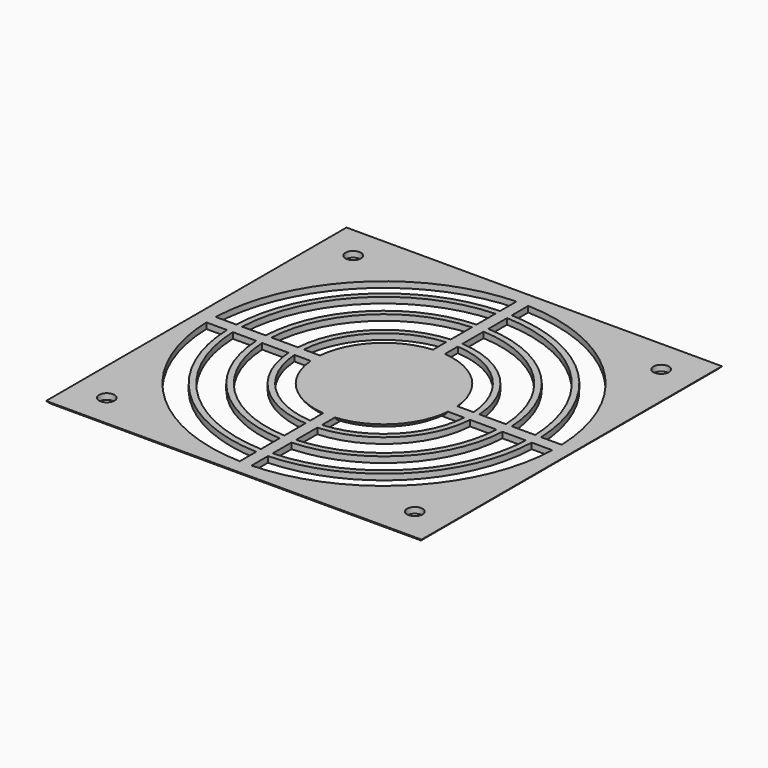
from build123d import *

# Parameters (mm, degrees)
F0_W            = 128
F0_H            = 128
F1_DEPTH        = 2
F3_DEPTH        = 25
F4_R            = 2.65
F5_DEPTH        = 25
F5_COPIES_COUNT = 4
F6_T1_DEPTH     = 148
F6_T3_DEPTH     = 148
F7_T4_ANGLE     = 122.478644554
F7_T9_ANGLE     = 122.478644554
F7_T15_ANGLE    = 122.478644554
F7_T20_ANGLE    = 122.478644554
F7_T25_ANGLE    = 122.478644554
F7_T31_ANGLE    = 122.478644554
F7_T36_ANGLE    = 122.478644554
F7_T41_ANGLE    = 122.478644554
F7_T47_ANGLE    = 122.478644554
F7_T52_ANGLE    = 122.478644554
F7_T57_ANGLE    = 122.478644554
F7_T63_ANGLE    = 122.478644554


# Not quite as in the source:
# - a fillet or chamfer that OpenCascade refuses, or shapes differently, is made with other operations: its cross-section is extruded or revolved along the edge and cut away or added
# - a pattern or mirror of a feature is missing from the dataset's text; its kind, count and spacing are read off the source's solid
# - a feature names something its author has since deleted; it is built from what else it names


with BuildPart() as f1:
    # F0 (on Top) → F1 (new body)
    with BuildSketch(Plane.XY):
        Rectangle(F0_W, F0_H)
    extrude(amount=F1_DEPTH)

    # F2 (on face) → F3 (cut)
    with BuildSketch(Plane.XY.offset(2)):
        with BuildLine():
            Line((51.9615242271, 2), (58.9660919512, 2))
            ThreePointArc((58.9660919512, 2), (41.71930009, 41.71930009), (2, 58.9660919512))
            Line((2, 58.9660919512), (2, 51.9615242271))
            ThreePointArc((2, 51.9615242271), (36.7695526217, 36.7695526217), (51.9615242271, 2))
        make_face()
        with BuildLine():
            Line((41.9523539268, 2), (49.9599839872, 2))
            ThreePointArc((49.9599839872, 2), (35.3553390593, 35.3553390593), (2, 49.9599839872))
            Line((2, 49.9599839872), (2, 41.9523539268))
            ThreePointArc((2, 41.9523539268), (29.6984848098, 29.6984848098), (41.9523539268, 2))
        make_face()
        with BuildLine():
            Line((30.9354165965, 2), (39.9499687109, 2))
            ThreePointArc((39.9499687109, 2), (28.2842712475, 28.2842712475), (2, 39.9499687109))
            Line((2, 39.9499687109), (2, 30.9354165965))
            ThreePointArc((2, 30.9354165965), (21.9203102168, 21.9203102168), (30.9354165965, 2))
        make_face()
        with BuildLine():
            Line((23.4147389479, 2), (28.930952283, 2))
            ThreePointArc((28.930952283, 2), (20.5060966544, 20.5060966544), (2, 28.930952283))
            Line((2, 28.930952283), (2, 23.4147389479))
            ThreePointArc((2, 23.4147389479), (16.6170093579, 16.6170093579), (23.4147389479, 2))
        make_face()
        with BuildLine():
            ThreePointArc((2, -28.930952283), (20.5060966544, -20.5060966544), (28.930952283, -2))
            Line((28.930952283, -2), (23.4147389479, -2))
            ThreePointArc((23.4147389479, -2), (16.6170093579, -16.6170093579), (2, -23.4147389479))
            Line((2, -23.4147389479), (2, -28.930952283))
        make_face()
        with BuildLine():
            ThreePointArc((2, -39.9499687109), (28.2842712475, -28.2842712475), (39.9499687109, -2))
            Line((39.9499687109, -2), (30.9354165965, -2))
            ThreePointArc((30.9354165965, -2), (21.9203102168, -21.9203102168), (2, -30.9354165965))
            Line((2, -30.9354165965), (2, -39.9499687109))
        make_face()
        with BuildLine():
            ThreePointArc((2, -49.9599839872), (35.3553390593, -35.3553390593), (49.9599839872, -2))
            Line((49.9599839872, -2), (41.9523539268, -2))
            ThreePointArc((41.9523539268, -2), (29.6984848098, -29.6984848098), (2, -41.9523539268))
            Line((2, -41.9523539268), (2, -49.9599839872))
        make_face()
        with BuildLine():
            ThreePointArc((2, -58.9660919512), (41.71930009, -41.71930009), (58.9660919512, -2))
            Line((58.9660919512, -2), (51.9615242271, -2))
            ThreePointArc((51.9615242271, -2), (36.7695526217, -36.7695526217), (2, -51.9615242271))
            Line((2, -51.9615242271), (2, -58.9660919512))
        make_face()
        with BuildLine():
            ThreePointArc((-28.930952283, -2), (-20.5060966544, -20.5060966544), (-2, -28.930952283))
            Line((-2, -28.930952283), (-2, -23.4147389479))
            ThreePointArc((-2, -23.4147389479), (-16.6170093579, -16.6170093579), (-23.4147389479, -2))
            Line((-23.4147389479, -2), (-28.930952283, -2))
        make_face()
        with BuildLine():
            ThreePointArc((-39.9499687109, -2), (-28.2842712475, -28.2842712475), (-2, -39.9499687109))
            Line((-2, -39.9499687109), (-2, -30.9354165965))
            ThreePointArc((-2, -30.9354165965), (-21.9203102168, -21.9203102168), (-30.9354165965, -2))
            Line((-30.9354165965, -2), (-39.9499687109, -2))
        make_face()
        with BuildLine():
            ThreePointArc((-49.9599839872, -2), (-35.3553390593, -35.3553390593), (-2, -49.9599839872))
            Line((-2, -49.9599839872), (-2, -41.9523539268))
            ThreePointArc((-2, -41.9523539268), (-29.6984848098, -29.6984848098), (-41.9523539268, -2))
            Line((-41.9523539268, -2), (-49.9599839872, -2))
        make_face()
        with BuildLine():
            ThreePointArc((-58.9660919512, -2), (-41.71930009, -41.71930009), (-2, -58.9660919512))
            Line((-2, -58.9660919512), (-2, -51.9615242271))
            ThreePointArc((-2, -51.9615242271), (-36.7695526217, -36.7695526217), (-51.9615242271, -2))
            Line((-51.9615242271, -2), (-58.9660919512, -2))
        make_face()
        with BuildLine():
            Line((-2, 23.4147389479), (-2, 28.930952283))
            ThreePointArc((-2, 28.930952283), (-20.5060966544, 20.5060966544), (-28.930952283, 2))
            Line((-28.930952283, 2), (-23.4147389479, 2))
            ThreePointArc((-23.4147389479, 2), (-16.6170093579, 16.6170093579), (-2, 23.4147389479))
        make_face()
        with BuildLine():
            Line((-2, 30.9354165965), (-2, 39.9499687109))
            ThreePointArc((-2, 39.9499687109), (-28.2842712475, 28.2842712475), (-39.9499687109, 2))
            Line((-39.9499687109, 2), (-30.9354165965, 2))
            ThreePointArc((-30.9354165965, 2), (-21.9203102168, 21.9203102168), (-2, 30.9354165965))
        make_face()
        with BuildLine():
            Line((-2, 41.9523539268), (-2, 49.9599839872))
            ThreePointArc((-2, 49.9599839872), (-35.3553390593, 35.3553390593), (-49.9599839872, 2))
            Line((-49.9599839872, 2), (-41.9523539268, 2))
            ThreePointArc((-41.9523539268, 2), (-29.6984848098, 29.6984848098), (-2, 41.9523539268))
        make_face()
        with BuildLine():
            Line((-2, 51.9615242271), (-2, 58.9660919512))
            ThreePointArc((-2, 58.9660919512), (-41.71930009, 41.71930009), (-58.9660919512, 2))
            Line((-58.9660919512, 2), (-51.9615242271, 2))
            ThreePointArc((-51.9615242271, 2), (-36.7695526217, 36.7695526217), (-2, 51.9615242271))
        make_face()
    extrude(amount=-F3_DEPTH, mode=Mode.SUBTRACT)

    # F4 (on face) → F5 (cut)
    with BuildSketch(Plane.XY.offset(2)):
        with Locations((-52.5, 52.5)):
            Circle(F4_R)
    f5 = extrude(amount=-F5_DEPTH, mode=Mode.SUBTRACT)

    # F5_copies: F5 ×4 about axis
    f5_copies_axis = Axis((0, 0, 0), (0, 0, 1))
    for i in range(1, F5_COPIES_COUNT):
        add(f5.rotate(f5_copies_axis, i * 360 / F5_COPIES_COUNT), mode=Mode.SUBTRACT)

    # F6: fillet of radius 5 on 4 edges, made by hand

    # F6_s2 → F6_t1 (cut)
    with BuildSketch(Plane.YZ.offset(-74)):
        with BuildLine():
            ThreePointArc((-60, 0), (-62.2360679775, 0.527864045), (-64, 2))
            Line((-64, 2), (-64, 0))
            Line((-64, 0), (-60, 0))
        make_face()
        with BuildLine():
            ThreePointArc((64, 2), (62.2360679775, 0.527864045), (60, 0))
            Line((60, 0), (64, 0))
            Line((64, 0), (64, 2))
        make_face()
    extrude(amount=F6_T1_DEPTH, mode=Mode.SUBTRACT)

    # F6_s4 → F6_t3 (cut)
    with BuildSketch(Plane.XZ.offset(-74)):
        with BuildLine():
            ThreePointArc((-64, 2), (-62.2360679775, 0.527864045), (-60, 0))
            Line((-60, 0), (-64, 0))
            Line((-64, 0), (-64, 2))
        make_face()
        with BuildLine():
            ThreePointArc((64, 2), (62.2360679775, 0.527864045), (60, 0))
            Line((60, 0), (64, 0))
            Line((64, 0), (64, 2))
        make_face()
    extrude(amount=F6_T3_DEPTH, mode=Mode.SUBTRACT)

    # F7: fillet of radius 4 on 4 edges, made by hand


with BuildPart() as f7_tool2:
    # F7_s3 → F7_t4 (revolve)
    with BuildSketch(Plane(origin=(0, 0, 0), x_dir=(0, 0, 1), z_dir=(0.960101987, -0.2796500929, 0))):
        with BuildLine():
            ThreePointArc((2, -23.5), (0.5358983849, -22.0358983849), (0, -20.0358983849))
            Line((0, -20.0358983849), (0, -23.5))
            Line((0, -23.5), (2, -23.5))
        make_face()
    revolve(axis=Axis((0, 0, 0), (0, 0, 1)), revolution_arc=F7_T4_ANGLE)

    split(bisect_by=Plane.YZ.offset(2), keep=Keep.TOP)


with BuildPart() as f1_1:
    add(f1.part)

    # F7_t1: cut F7_tool2
    add(f7_tool2.part, mode=Mode.SUBTRACT)


with BuildPart() as f7_tool7:
    # F7_s8 → F7_t9 (revolve)
    with BuildSketch(Plane(origin=(0, 0, 0), x_dir=(0, 0, 1), z_dir=(0.960101987, -0.2796500929, 0))):
        with BuildLine():
            ThreePointArc((2, -23.5), (0.5358983849, -22.0358983849), (0, -20.0358983849))
            Line((0, -20.0358983849), (0, -23.5))
            Line((0, -23.5), (2, -23.5))
        make_face()
    revolve(axis=Axis((0, 0, 0), (0, 0, 1)), revolution_arc=F7_T9_ANGLE)

    split(bisect_by=Plane.YZ.offset(-2), keep=Keep.BOTTOM)

    split(bisect_by=Plane.XZ.offset(-2), keep=Keep.BOTTOM)


with BuildPart() as f1_2:
    add(f1_1.part)

    # F7_t6: cut F7_tool7
    add(f7_tool7.part, mode=Mode.SUBTRACT)


with BuildPart() as f7_tool13:
    # F7_s14 → F7_t15 (revolve)
    with BuildSketch(Plane(origin=(0, 0, 0), x_dir=(0, 0, 1), z_dir=(0.960101987, -0.2796500929, 0))):
        with BuildLine():
            ThreePointArc((2, -23.5), (0.5358983849, -22.0358983849), (0, -20.0358983849))
            Line((0, -20.0358983849), (0, -23.5))
            Line((0, -23.5), (2, -23.5))
        make_face()
    revolve(axis=Axis((0, 0, 0), (0, 0, 1)), revolution_arc=F7_T15_ANGLE)

    split(bisect_by=Plane.XZ.offset(2), keep=Keep.TOP)


with BuildPart() as f1_3:
    add(f1_2.part)

    # F7_t12: cut F7_tool13
    add(f7_tool13.part, mode=Mode.SUBTRACT)


with BuildPart() as f7_tool18:
    # F7_s19 → F7_t20 (revolve)
    with BuildSketch(Plane(origin=(0, 0, 0), x_dir=(0, 0, 1), z_dir=(-0.2796500929, -0.960101987, 0))):
        with BuildLine():
            ThreePointArc((2, -23.5), (0.5358983849, -22.0358983849), (0, -20.0358983849))
            Line((0, -20.0358983849), (0, -23.5))
            Line((0, -23.5), (2, -23.5))
        make_face()
    revolve(axis=Axis((0, 0, 0), (0, 0, 1)), revolution_arc=F7_T20_ANGLE)

    split(bisect_by=Plane.XZ.offset(2), keep=Keep.TOP)


with BuildPart() as f1_4:
    add(f1_3.part)

    # F7_t17: cut F7_tool18
    add(f7_tool18.part, mode=Mode.SUBTRACT)


with BuildPart() as f7_tool23:
    # F7_s24 → F7_t25 (revolve)
    with BuildSketch(Plane(origin=(0, 0, 0), x_dir=(0, 0, 1), z_dir=(-0.2796500929, -0.960101987, 0))):
        with BuildLine():
            ThreePointArc((2, -23.5), (0.5358983849, -22.0358983849), (0, -20.0358983849))
            Line((0, -20.0358983849), (0, -23.5))
            Line((0, -23.5), (2, -23.5))
        make_face()
    revolve(axis=Axis((0, 0, 0), (0, 0, 1)), revolution_arc=F7_T25_ANGLE)

    split(bisect_by=Plane.XZ.offset(-2), keep=Keep.BOTTOM)

    split(bisect_by=Plane.YZ.offset(2), keep=Keep.TOP)


with BuildPart() as f1_5:
    add(f1_4.part)

    # F7_t22: cut F7_tool23
    add(f7_tool23.part, mode=Mode.SUBTRACT)


with BuildPart() as f7_tool29:
    # F7_s30 → F7_t31 (revolve)
    with BuildSketch(Plane(origin=(0, 0, 0), x_dir=(0, 0, 1), z_dir=(-0.2796500929, -0.960101987, 0))):
        with BuildLine():
            ThreePointArc((2, -23.5), (0.5358983849, -22.0358983849), (0, -20.0358983849))
            Line((0, -20.0358983849), (0, -23.5))
            Line((0, -23.5), (2, -23.5))
        make_face()
    revolve(axis=Axis((0, 0, 0), (0, 0, 1)), revolution_arc=F7_T31_ANGLE)

    split(bisect_by=Plane.YZ.offset(-2), keep=Keep.BOTTOM)


with BuildPart() as f1_6:
    add(f1_5.part)

    # F7_t28: cut F7_tool29
    add(f7_tool29.part, mode=Mode.SUBTRACT)


with BuildPart() as f7_tool34:
    # F7_s35 → F7_t36 (revolve)
    with BuildSketch(Plane(origin=(0, 0, 0), x_dir=(0, 0, 1), z_dir=(-0.960101987, 0.2796500929, 0))):
        with BuildLine():
            ThreePointArc((2, -23.5), (0.5358983849, -22.0358983849), (0, -20.0358983849))
            Line((0, -20.0358983849), (0, -23.5))
            Line((0, -23.5), (2, -23.5))
        make_face()
    revolve(axis=Axis((0, 0, 0), (0, 0, 1)), revolution_arc=F7_T36_ANGLE)

    split(bisect_by=Plane.YZ.offset(-2), keep=Keep.BOTTOM)


with BuildPart() as f1_7:
    add(f1_6.part)

    # F7_t33: cut F7_tool34
    add(f7_tool34.part, mode=Mode.SUBTRACT)


with BuildPart() as f7_tool39:
    # F7_s40 → F7_t41 (revolve)
    with BuildSketch(Plane(origin=(0, 0, 0), x_dir=(0, 0, 1), z_dir=(-0.960101987, 0.2796500929, 0))):
        with BuildLine():
            ThreePointArc((2, -23.5), (0.5358983849, -22.0358983849), (0, -20.0358983849))
            Line((0, -20.0358983849), (0, -23.5))
            Line((0, -23.5), (2, -23.5))
        make_face()
    revolve(axis=Axis((0, 0, 0), (0, 0, 1)), revolution_arc=F7_T41_ANGLE)

    split(bisect_by=Plane.XZ.offset(2), keep=Keep.TOP)

    split(bisect_by=Plane.YZ.offset(2), keep=Keep.TOP)


with BuildPart() as f1_8:
    add(f1_7.part)

    # F7_t38: cut F7_tool39
    add(f7_tool39.part, mode=Mode.SUBTRACT)


with BuildPart() as f7_tool45:
    # F7_s46 → F7_t47 (revolve)
    with BuildSketch(Plane(origin=(0, 0, 0), x_dir=(0, 0, 1), z_dir=(-0.960101987, 0.2796500929, 0))):
        with BuildLine():
            ThreePointArc((2, -23.5), (0.5358983849, -22.0358983849), (0, -20.0358983849))
            Line((0, -20.0358983849), (0, -23.5))
            Line((0, -23.5), (2, -23.5))
        make_face()
    revolve(axis=Axis((0, 0, 0), (0, 0, 1)), revolution_arc=F7_T47_ANGLE)

    split(bisect_by=Plane.XZ.offset(-2), keep=Keep.BOTTOM)


with BuildPart() as f1_9:
    add(f1_8.part)

    # F7_t44: cut F7_tool45
    add(f7_tool45.part, mode=Mode.SUBTRACT)


with BuildPart() as f7_tool50:
    # F7_s51 → F7_t52 (revolve)
    with BuildSketch(Plane(origin=(0, 0, 0), x_dir=(0, 0, 1), z_dir=(0.2796500929, 0.960101987, 0))):
        with BuildLine():
            ThreePointArc((2, -23.5), (0.5358983849, -22.0358983849), (0, -20.0358983849))
            Line((0, -20.0358983849), (0, -23.5))
            Line((0, -23.5), (2, -23.5))
        make_face()
    revolve(axis=Axis((0, 0, 0), (0, 0, 1)), revolution_arc=F7_T52_ANGLE)

    split(bisect_by=Plane.XZ.offset(-2), keep=Keep.BOTTOM)


with BuildPart() as f1_10:
    add(f1_9.part)

    # F7_t49: cut F7_tool50
    add(f7_tool50.part, mode=Mode.SUBTRACT)


with BuildPart() as f7_tool55:
    # F7_s56 → F7_t57 (revolve)
    with BuildSketch(Plane(origin=(0, 0, 0), x_dir=(0, 0, 1), z_dir=(0.2796500929, 0.960101987, 0))):
        with BuildLine():
            ThreePointArc((2, -23.5), (0.5358983849, -22.0358983849), (0, -20.0358983849))
            Line((0, -20.0358983849), (0, -23.5))
            Line((0, -23.5), (2, -23.5))
        make_face()
    revolve(axis=Axis((0, 0, 0), (0, 0, 1)), revolution_arc=F7_T57_ANGLE)

    split(bisect_by=Plane.YZ.offset(-2), keep=Keep.BOTTOM)

    split(bisect_by=Plane.XZ.offset(2), keep=Keep.TOP)


with BuildPart() as f1_11:
    add(f1_10.part)

    # F7_t54: cut F7_tool55
    add(f7_tool55.part, mode=Mode.SUBTRACT)


with BuildPart() as f7_tool61:
    # F7_s62 → F7_t63 (revolve)
    with BuildSketch(Plane(origin=(0, 0, 0), x_dir=(0, 0, 1), z_dir=(0.2796500929, 0.960101987, 0))):
        with BuildLine():
            ThreePointArc((2, -23.5), (0.5358983849, -22.0358983849), (0, -20.0358983849))
            Line((0, -20.0358983849), (0, -23.5))
            Line((0, -23.5), (2, -23.5))
        make_face()
    revolve(axis=Axis((0, 0, 0), (0, 0, 1)), revolution_arc=F7_T63_ANGLE)

    split(bisect_by=Plane.YZ.offset(2), keep=Keep.TOP)


with BuildPart() as f1_12:
    add(f1_11.part)

    # F7_t60: cut F7_tool61
    add(f7_tool61.part, mode=Mode.SUBTRACT)


solid = f1_12.part
